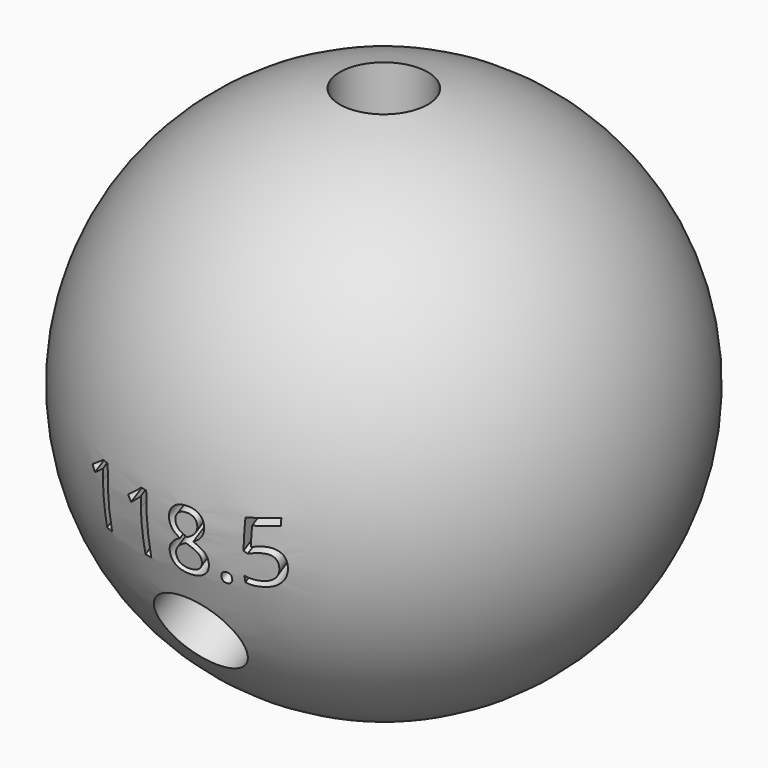
from build123d import *

# Parameters (mm, degrees)
F5_R          = 3.175
F6_DEPTH      = 76.2
F7_ANGLE      = 118.5
F8_ANGLE      = 119.8
F10_TEXT_SIZE = 5.7784387738
F11_DEPTH     = 6.35
F13_TEXT_SIZE = 6.645384969
F14_DEPTH     = 6.35


# Not quite as in the source:
# - Text() gives the source's letters only with a copy of the font that has no kerning and outlines rounded to 1/6400 em; it was checked with that copy


with BuildPart() as f2:
    # F0 (on Front) → F2 (revolve)
    with BuildSketch(Plane.XZ):
        with BuildLine():
            Line((0, -19.05), (0, 19.05))
            ThreePointArc((0, 19.05), (-19.05, 0), (0, -19.05))
        make_face()
    revolve(axis=Axis((0, 0, 0), (0, 0, 1)))

    # F10 (on offset) → F11 (cut)
    with BuildSketch(Plane(origin=(0, -17.8575637293, -9.6958660085), x_dir=(1, 0, 0), z_dir=(0, -0.8788171127, -0.4771587603))):
        with Locations((-7.3158596642, 5.1700836048)):
            Text('118.5', F10_TEXT_SIZE, font='Open Sans', text_align=(TextAlign.LEFT, TextAlign.BOTTOM))
    extrude(amount=-F11_DEPTH, mode=Mode.SUBTRACT)

    # F13 (on offset) → F14 (cut)
    with BuildSketch(Plane(origin=(0, 17.2884817435, -10.6775839498), x_dir=(-1, 0, 0), z_dir=(0, 0.8508111094, -0.5254716511))):
        with Locations((-8.5263404176, 4.5956606045)):
            Text('119.8', F13_TEXT_SIZE, font='Open Sans', text_align=(TextAlign.LEFT, TextAlign.BOTTOM))
    extrude(amount=-F14_DEPTH, mode=Mode.SUBTRACT)


with BuildPart() as f6:
    # F5 (on offset) → F6 (new body)
    with BuildSketch(Plane.XY.offset(7.62)):
        Circle(F5_R)
    extrude(amount=F6_DEPTH)


with BuildPart() as f7_1:
    # F7: copy of F6
    add(f6.part.rotate(Axis((38.1614528596, 0, 0), (1, 0, 0)), F7_ANGLE))


with BuildPart() as f8_1:
    # F8: copy of F7_1
    add(f7_1.part.rotate(Axis((38.1614528596, 0, 0), (1, 0, 0)), F8_ANGLE))


with BuildPart() as f2_1:
    add(f2.part)

    # F15: cut F6, F7_1, F8_1
    add(f6.part, mode=Mode.SUBTRACT)
    add(f7_1.part, mode=Mode.SUBTRACT)
    add(f8_1.part, mode=Mode.SUBTRACT)


solid = f2_1.part
